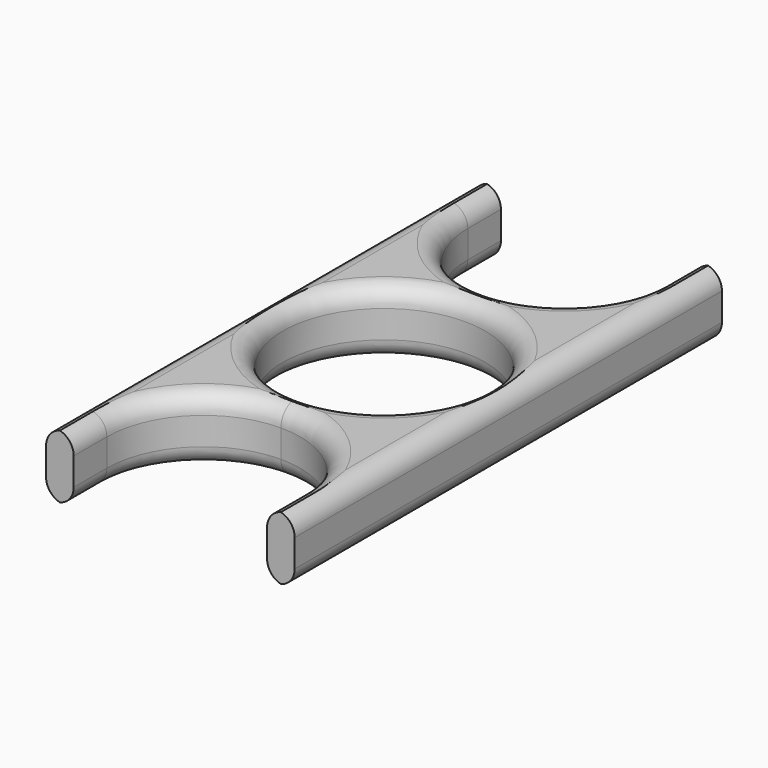
from build123d import *

# Parameters (mm, degrees)
F0_R          = 11
F1_DEPTH      = 7
F2_R          = 10.49999
F3_T1_DEPTH   = 9.50001
F3_T3_DEPTH   = 2e-05
F3_T5_DEPTH   = 68
F3_T7_DEPTH   = 9.50001
F3_T10_ANGLE  = 90
F3_T14_DEPTH  = 13
F3_S15_R      = 2
F3_T16_DEPTH  = 8
F3_T20_DEPTH  = 13
F3_S21_R      = 2
F3_T22_DEPTH  = 8
F3_T24_ANGLE  = 90
F3_T28_DEPTH  = 13
F3_S29_R      = 2
F3_T30_DEPTH  = 8
F3_T34_DEPTH  = 13
F3_S35_R      = 2
F3_T36_DEPTH  = 8
F3_T40_DEPTH  = 13
F3_S41_R      = 2
F3_T42_DEPTH  = 8
F3_T46_DEPTH  = 13
F3_S47_R      = 2
F3_T48_DEPTH  = 8
F3_T50_ANGLE  = 90
F3_T54_DEPTH  = 13
F3_S55_R      = 2
F3_T56_DEPTH  = 8
F3_T60_DEPTH  = 13
F3_S61_R      = 2
F3_T62_DEPTH  = 8
F3_T64_ANGLE  = 90
F3_T68_ANGLE  = 90
F3_T72_DEPTH  = 13
F3_S73_R      = 2
F3_T74_DEPTH  = 8
F3_T78_DEPTH  = 13
F3_S79_R      = 2
F3_T80_DEPTH  = 8
F3_T82_ANGLE  = 90
F3_T86_DEPTH  = 13
F3_S87_R      = 2
F3_T88_DEPTH  = 8
F3_T92_DEPTH  = 13
F3_S93_R      = 2
F3_T94_DEPTH  = 8
F3_T98_DEPTH  = 13
F3_S99_R      = 2
F3_T100_DEPTH = 8
F3_T104_DEPTH = 13
F3_S105_R     = 2
F3_T106_DEPTH = 8
F3_T108_ANGLE = 90
F3_T112_DEPTH = 13
F3_S113_R     = 2
F3_T114_DEPTH = 8
F3_T118_DEPTH = 13
F3_S119_R     = 2
F3_T120_DEPTH = 8
F3_T122_ANGLE = 90


# Not quite as in the source:
# - a fillet or chamfer that OpenCascade refuses, or shapes differently, is made with other operations: its cross-section is extruded or revolved along the edge and cut away or added
# - a fillet or chamfer is up to 0.001 mm smaller than in the source, because OpenCascade refuses the exact size


with BuildPart() as f1:
    # F0 (on Top) → F1 (new body)
    with BuildSketch(Plane.XY):
        Polygon((13.5, -29), (13.5, 29), (10.5, 29), (10.5, 14), (-10.5, 14), (-10.5, 29), (-13.5, 29), (-13.5, -29), (-10.5, -29), (-10.5, -14), (10.5, -14), (10.5, -29), align=None)
        Circle(F0_R, mode=Mode.SUBTRACT)
    extrude(amount=F1_DEPTH)

    # F2 (radius 10.5 in the source; OpenCascade refuses exactly that, so slightly less here)
    f2_edges = [f1.edges().sort_by_distance(p)[0] for p in [
        (-10.5, -14, 3.5),
        (10.5, -14, 3.5),
        (-10.5, 14, 3.5),
        (10.5, 14, 3.5),
    ]]
    fillet(f2_edges, radius=F2_R)

    # F3: fillet of radius 2 on 34 edges, made by hand

    # F3_s2 → F3_t1 (cut)
    with BuildSketch(Plane.XZ.offset(-34)):
        with BuildLine():
            ThreePointArc((10.5, 5), (11.0857864376, 6.4142135624), (12.5, 7))
            Line((12.5, 7), (10.5, 7))
            Line((10.5, 7), (10.5, 5))
        make_face()
        with BuildLine():
            ThreePointArc((-12.5, 7), (-11.0857864376, 6.4142135624), (-10.5, 5))
            Line((-10.5, 5), (-10.5, 7))
            Line((-10.5, 7), (-12.5, 7))
        make_face()
        with BuildLine():
            ThreePointArc((10.5, 2), (11.0857864376, 0.5857864376), (12.5, 0))
            Line((12.5, 0), (10.5, 0))
            Line((10.5, 0), (10.5, 2))
        make_face()
        with BuildLine():
            ThreePointArc((-12.5, 0), (-11.0857864376, 0.5857864376), (-10.5, 2))
            Line((-10.5, 2), (-10.5, 0))
            Line((-10.5, 0), (-12.5, 0))
        make_face()
    extrude(amount=F3_T1_DEPTH, mode=Mode.SUBTRACT)

    # F3_s4 → F3_t3 (cut)
    with BuildSketch(Plane.YZ.offset(-1e-05)):
        with BuildLine():
            ThreePointArc((12, 7), (13.4142135624, 6.4142135624), (14, 5))
            Line((14, 5), (14, 7))
            Line((14, 7), (12, 7))
        make_face()
        with BuildLine():
            ThreePointArc((-12, 7), (-13.4142135624, 6.4142135624), (-14, 5))
            Line((-14, 5), (-14, 7))
            Line((-14, 7), (-12, 7))
        make_face()
        with BuildLine():
            ThreePointArc((12, 0), (13.4142135624, 0.5857864376), (14, 2))
            Line((14, 2), (14, 0))
            Line((14, 0), (12, 0))
        make_face()
        with BuildLine():
            ThreePointArc((-12, 0), (-13.4142135624, 0.5857864376), (-14, 2))
            Line((-14, 2), (-14, 0))
            Line((-14, 0), (-12, 0))
        make_face()
    extrude(amount=F3_T3_DEPTH, mode=Mode.SUBTRACT)

    # F3_s6 → F3_t5 (cut)
    with BuildSketch(Plane.XZ.offset(-34)):
        with BuildLine():
            ThreePointArc((11.5, 7), (12.9142135624, 6.4142135624), (13.5, 5))
            Line((13.5, 5), (13.5, 7))
            Line((13.5, 7), (11.5, 7))
        make_face()
        with BuildLine():
            ThreePointArc((-11.5, 7), (-12.9142135624, 6.4142135624), (-13.5, 5))
            Line((-13.5, 5), (-13.5, 7))
            Line((-13.5, 7), (-11.5, 7))
        make_face()
        with BuildLine():
            ThreePointArc((11.5, 0), (12.9142135624, 0.5857864376), (13.5, 2))
            Line((13.5, 2), (13.5, 0))
            Line((13.5, 0), (11.5, 0))
        make_face()
        with BuildLine():
            ThreePointArc((-11.5, 0), (-12.9142135624, 0.5857864376), (-13.5, 2))
            Line((-13.5, 2), (-13.5, 0))
            Line((-13.5, 0), (-11.5, 0))
        make_face()
    extrude(amount=F3_T5_DEPTH, mode=Mode.SUBTRACT)

    # F3_s8 → F3_t7 (cut)
    with BuildSketch(Plane.XZ.offset(24.49999)):
        with BuildLine():
            ThreePointArc((12.5, 7), (11.0857864376, 6.4142135624), (10.5, 5))
            Line((10.5, 5), (10.5, 7))
            Line((10.5, 7), (12.5, 7))
        make_face()
        with BuildLine():
            ThreePointArc((-12.5, 7), (-11.0857864376, 6.4142135624), (-10.5, 5))
            Line((-10.5, 5), (-10.5, 7))
            Line((-10.5, 7), (-12.5, 7))
        make_face()
        with BuildLine():
            ThreePointArc((12.5, 0), (11.0857864376, 0.5857864376), (10.5, 2))
            Line((10.5, 2), (10.5, 0))
            Line((10.5, 0), (12.5, 0))
        make_face()
        with BuildLine():
            ThreePointArc((-12.5, 0), (-11.0857864376, 0.5857864376), (-10.5, 2))
            Line((-10.5, 2), (-10.5, 0))
            Line((-10.5, 0), (-12.5, 0))
        make_face()
    extrude(amount=F3_T7_DEPTH, mode=Mode.SUBTRACT)

    # F3_s9 → F3_t10 (revolve, cut)
    with BuildSketch(Plane.XZ.offset(-24.49999)):
        with BuildLine():
            ThreePointArc((10.5, 5), (11.0857864376, 6.4142135624), (12.5, 7))
            Line((12.5, 7), (10.5, 7))
            Line((10.5, 7), (10.5, 5))
        make_face()
    revolve(axis=Axis((1e-05, 24.49999, 7), (0, 0, -1)), revolution_arc=F3_T10_ANGLE, mode=Mode.SUBTRACT)


with BuildPart() as f3_tool12:
    # F3_s13 → F3_t14 (new body)
    with BuildSketch(Plane.YZ.offset(18.5)):
        with BuildLine():
            ThreePointArc((29, 5), (28.4142135624, 6.4142135624), (27, 7))
            Line((27, 7), (29, 7))
            Line((29, 7), (29, 5))
        make_face()
    extrude(amount=-F3_T14_DEPTH)

    # F3_s15 → F3_t16 (cut, symmetric)
    with BuildSketch(Plane.XZ.offset(-28)):
        with Locations((12.5, 5)):
            Circle(F3_S15_R)
    extrude(amount=F3_T16_DEPTH, both=True, mode=Mode.SUBTRACT)


with BuildPart() as f1_1:
    add(f1.part)

    # F3_t11: cut F3_tool12
    add(f3_tool12.part, mode=Mode.SUBTRACT)


with BuildPart() as f3_tool18:
    # F3_s19 → F3_t20 (new body)
    with BuildSketch(Plane.YZ.offset(18.5)):
        with BuildLine():
            ThreePointArc((29, 5), (28.4142135624, 6.4142135624), (27, 7))
            Line((27, 7), (29, 7))
            Line((29, 7), (29, 5))
        make_face()
    extrude(amount=-F3_T20_DEPTH)

    # F3_s21 → F3_t22 (cut, symmetric)
    with BuildSketch(Plane.XZ.offset(-28)):
        with Locations((11.5, 5)):
            Circle(F3_S21_R)
    extrude(amount=F3_T22_DEPTH, both=True, mode=Mode.SUBTRACT)


with BuildPart() as f1_2:
    add(f1_1.part)

    # F3_t17: cut F3_tool18
    add(f3_tool18.part, mode=Mode.SUBTRACT)

    # F3_s23 → F3_t24 (revolve, cut)
    with BuildSketch(Plane.YZ.offset(-1e-05)):
        with BuildLine():
            ThreePointArc((12, 7), (13.4142135624, 6.4142135624), (14, 5))
            Line((14, 5), (14, 7))
            Line((14, 7), (12, 7))
        make_face()
    revolve(axis=Axis((-1e-05, 24.49999, 7), (0, 0, -1)), revolution_arc=F3_T24_ANGLE, mode=Mode.SUBTRACT)


with BuildPart() as f3_tool26:
    # F3_s27 → F3_t28 (new body)
    with BuildSketch(Plane.YZ.offset(5.5)):
        with BuildLine():
            ThreePointArc((-27, 7), (-28.4142135624, 6.4142135624), (-29, 5))
            Line((-29, 5), (-29, 7))
            Line((-29, 7), (-27, 7))
        make_face()
    extrude(amount=F3_T28_DEPTH)

    # F3_s29 → F3_t30 (cut, symmetric)
    with BuildSketch(Plane.XZ.offset(28)):
        with Locations((12.5, 5)):
            Circle(F3_S29_R)
    extrude(amount=F3_T30_DEPTH, both=True, mode=Mode.SUBTRACT)


with BuildPart() as f1_3:
    add(f1_2.part)

    # F3_t25: cut F3_tool26
    add(f3_tool26.part, mode=Mode.SUBTRACT)


with BuildPart() as f3_tool32:
    # F3_s33 → F3_t34 (new body)
    with BuildSketch(Plane.YZ.offset(5.5)):
        with BuildLine():
            ThreePointArc((-27, 7), (-28.4142135624, 6.4142135624), (-29, 5))
            Line((-29, 5), (-29, 7))
            Line((-29, 7), (-27, 7))
        make_face()
    extrude(amount=F3_T34_DEPTH)

    # F3_s35 → F3_t36 (cut, symmetric)
    with BuildSketch(Plane.XZ.offset(28)):
        with Locations((11.5, 5)):
            Circle(F3_S35_R)
    extrude(amount=F3_T36_DEPTH, both=True, mode=Mode.SUBTRACT)


with BuildPart() as f1_4:
    add(f1_3.part)

    # F3_t31: cut F3_tool32
    add(f3_tool32.part, mode=Mode.SUBTRACT)


with BuildPart() as f3_tool38:
    # F3_s39 → F3_t40 (new body)
    with BuildSketch(Plane.YZ.offset(-5.5)):
        with BuildLine():
            ThreePointArc((27, 7), (28.4142135624, 6.4142135624), (29, 5))
            Line((29, 5), (29, 7))
            Line((29, 7), (27, 7))
        make_face()
    extrude(amount=-F3_T40_DEPTH)

    # F3_s41 → F3_t42 (cut, symmetric)
    with BuildSketch(Plane.XZ.offset(-28)):
        with Locations((-12.5, 5)):
            Circle(F3_S41_R)
    extrude(amount=F3_T42_DEPTH, both=True, mode=Mode.SUBTRACT)


with BuildPart() as f1_5:
    add(f1_4.part)

    # F3_t37: cut F3_tool38
    add(f3_tool38.part, mode=Mode.SUBTRACT)


with BuildPart() as f3_tool44:
    # F3_s45 → F3_t46 (new body)
    with BuildSketch(Plane.YZ.offset(-5.5)):
        with BuildLine():
            ThreePointArc((27, 7), (28.4142135624, 6.4142135624), (29, 5))
            Line((29, 5), (29, 7))
            Line((29, 7), (27, 7))
        make_face()
    extrude(amount=-F3_T46_DEPTH)

    # F3_s47 → F3_t48 (cut, symmetric)
    with BuildSketch(Plane.XZ.offset(-28)):
        with Locations((-11.5, 5)):
            Circle(F3_S47_R)
    extrude(amount=F3_T48_DEPTH, both=True, mode=Mode.SUBTRACT)


with BuildPart() as f1_6:
    add(f1_5.part)

    # F3_t43: cut F3_tool44
    add(f3_tool44.part, mode=Mode.SUBTRACT)

    # F3_s49 → F3_t50 (revolve, cut)
    with BuildSketch(Plane.YZ.offset(1e-05)):
        with BuildLine():
            ThreePointArc((-12, 7), (-13.4142135624, 6.4142135624), (-14, 5))
            Line((-14, 5), (-14, 7))
            Line((-14, 7), (-12, 7))
        make_face()
    revolve(axis=Axis((1e-05, -24.49999, 7), (0, 0, -1)), revolution_arc=F3_T50_ANGLE, mode=Mode.SUBTRACT)


with BuildPart() as f3_tool52:
    # F3_s53 → F3_t54 (new body)
    with BuildSketch(Plane.YZ.offset(-18.5)):
        with BuildLine():
            ThreePointArc((-27, 7), (-28.4142135624, 6.4142135624), (-29, 5))
            Line((-29, 5), (-29, 7))
            Line((-29, 7), (-27, 7))
        make_face()
    extrude(amount=F3_T54_DEPTH)

    # F3_s55 → F3_t56 (cut, symmetric)
    with BuildSketch(Plane.XZ.offset(28)):
        with Locations((-12.5, 5)):
            Circle(F3_S55_R)
    extrude(amount=F3_T56_DEPTH, both=True, mode=Mode.SUBTRACT)


with BuildPart() as f1_7:
    add(f1_6.part)

    # F3_t51: cut F3_tool52
    add(f3_tool52.part, mode=Mode.SUBTRACT)


with BuildPart() as f3_tool58:
    # F3_s59 → F3_t60 (new body)
    with BuildSketch(Plane.YZ.offset(-18.5)):
        with BuildLine():
            ThreePointArc((-27, 7), (-28.4142135624, 6.4142135624), (-29, 5))
            Line((-29, 5), (-29, 7))
            Line((-29, 7), (-27, 7))
        make_face()
    extrude(amount=F3_T60_DEPTH)

    # F3_s61 → F3_t62 (cut, symmetric)
    with BuildSketch(Plane.XZ.offset(28)):
        with Locations((-11.5, 5)):
            Circle(F3_S61_R)
    extrude(amount=F3_T62_DEPTH, both=True, mode=Mode.SUBTRACT)


with BuildPart() as f1_8:
    add(f1_7.part)

    # F3_t57: cut F3_tool58
    add(f3_tool58.part, mode=Mode.SUBTRACT)

    # F3_s63 → F3_t64 (revolve, cut)
    with BuildSketch(Plane.XZ.offset(24.49999)):
        with BuildLine():
            ThreePointArc((-12.5, 7), (-11.0857864376, 6.4142135624), (-10.5, 5))
            Line((-10.5, 5), (-10.5, 7))
            Line((-10.5, 7), (-12.5, 7))
        make_face()
    revolve(axis=Axis((-1e-05, -24.49999, 7), (0, 0, -1)), revolution_arc=F3_T64_ANGLE, mode=Mode.SUBTRACT)

    # F3_s65 → F3_t66 (revolve, cut)
    with BuildSketch(Plane.XZ):
        with BuildLine():
            ThreePointArc((13, 7), (11.5857864376, 6.4142135624), (11, 5))
            Line((11, 5), (11, 7))
            Line((11, 7), (13, 7))
        make_face()
    revolve(axis=Axis((0, 0, 7), (0, 0, 1)), mode=Mode.SUBTRACT)

    # F3_s67 → F3_t68 (revolve, cut)
    with BuildSketch(Plane.XZ.offset(-24.49999)):
        with BuildLine():
            ThreePointArc((12.5, 0), (11.0857864376, 0.5857864376), (10.5, 2))
            Line((10.5, 2), (10.5, 0))
            Line((10.5, 0), (12.5, 0))
        make_face()
    revolve(axis=Axis((1e-05, 24.49999, 0), (0, 0, -1)), revolution_arc=F3_T68_ANGLE, mode=Mode.SUBTRACT)


with BuildPart() as f3_tool70:
    # F3_s71 → F3_t72 (new body)
    with BuildSketch(Plane.YZ.offset(18.5)):
        with BuildLine():
            ThreePointArc((27, 0), (28.4142135624, 0.5857864376), (29, 2))
            Line((29, 2), (29, 0))
            Line((29, 0), (27, 0))
        make_face()
    extrude(amount=-F3_T72_DEPTH)

    # F3_s73 → F3_t74 (cut, symmetric)
    with BuildSketch(Plane.XZ.offset(-28)):
        with Locations((11.5, 2)):
            Circle(F3_S73_R)
    extrude(amount=F3_T74_DEPTH, both=True, mode=Mode.SUBTRACT)


with BuildPart() as f1_9:
    add(f1_8.part)

    # F3_t69: cut F3_tool70
    add(f3_tool70.part, mode=Mode.SUBTRACT)


with BuildPart() as f3_tool76:
    # F3_s77 → F3_t78 (new body)
    with BuildSketch(Plane.YZ.offset(18.5)):
        with BuildLine():
            ThreePointArc((27, 0), (28.4142135624, 0.5857864376), (29, 2))
            Line((29, 2), (29, 0))
            Line((29, 0), (27, 0))
        make_face()
    extrude(amount=-F3_T78_DEPTH)

    # F3_s79 → F3_t80 (cut, symmetric)
    with BuildSketch(Plane.XZ.offset(-28)):
        with Locations((12.5, 2)):
            Circle(F3_S79_R)
    extrude(amount=F3_T80_DEPTH, both=True, mode=Mode.SUBTRACT)


with BuildPart() as f1_10:
    add(f1_9.part)

    # F3_t75: cut F3_tool76
    add(f3_tool76.part, mode=Mode.SUBTRACT)

    # F3_s81 → F3_t82 (revolve, cut)
    with BuildSketch(Plane.YZ.offset(-1e-05)):
        with BuildLine():
            ThreePointArc((12, 0), (13.4142135624, 0.5857864376), (14, 2))
            Line((14, 2), (14, 0))
            Line((14, 0), (12, 0))
        make_face()
    revolve(axis=Axis((-1e-05, 24.49999, 0), (0, 0, -1)), revolution_arc=F3_T82_ANGLE, mode=Mode.SUBTRACT)


with BuildPart() as f3_tool84:
    # F3_s85 → F3_t86 (new body)
    with BuildSketch(Plane.YZ.offset(5.5)):
        with BuildLine():
            ThreePointArc((-27, 0), (-28.4142135624, 0.5857864376), (-29, 2))
            Line((-29, 2), (-29, 0))
            Line((-29, 0), (-27, 0))
        make_face()
    extrude(amount=F3_T86_DEPTH)

    # F3_s87 → F3_t88 (cut, symmetric)
    with BuildSketch(Plane.XZ.offset(28)):
        with Locations((11.5, 2)):
            Circle(F3_S87_R)
    extrude(amount=F3_T88_DEPTH, both=True, mode=Mode.SUBTRACT)


with BuildPart() as f1_11:
    add(f1_10.part)

    # F3_t83: cut F3_tool84
    add(f3_tool84.part, mode=Mode.SUBTRACT)


with BuildPart() as f3_tool90:
    # F3_s91 → F3_t92 (new body)
    with BuildSketch(Plane.YZ.offset(5.5)):
        with BuildLine():
            ThreePointArc((-27, 0), (-28.4142135624, 0.5857864376), (-29, 2))
            Line((-29, 2), (-29, 0))
            Line((-29, 0), (-27, 0))
        make_face()
    extrude(amount=F3_T92_DEPTH)

    # F3_s93 → F3_t94 (cut, symmetric)
    with BuildSketch(Plane.XZ.offset(28)):
        with Locations((12.5, 2)):
            Circle(F3_S93_R)
    extrude(amount=F3_T94_DEPTH, both=True, mode=Mode.SUBTRACT)


with BuildPart() as f1_12:
    add(f1_11.part)

    # F3_t89: cut F3_tool90
    add(f3_tool90.part, mode=Mode.SUBTRACT)


with BuildPart() as f3_tool96:
    # F3_s97 → F3_t98 (new body)
    with BuildSketch(Plane.YZ.offset(-5.5)):
        with BuildLine():
            ThreePointArc((27, 0), (28.4142135624, 0.5857864376), (29, 2))
            Line((29, 2), (29, 0))
            Line((29, 0), (27, 0))
        make_face()
    extrude(amount=-F3_T98_DEPTH)

    # F3_s99 → F3_t100 (cut, symmetric)
    with BuildSketch(Plane.XZ.offset(-28)):
        with Locations((-11.5, 2)):
            Circle(F3_S99_R)
    extrude(amount=F3_T100_DEPTH, both=True, mode=Mode.SUBTRACT)


with BuildPart() as f1_13:
    add(f1_12.part)

    # F3_t95: cut F3_tool96
    add(f3_tool96.part, mode=Mode.SUBTRACT)


with BuildPart() as f3_tool102:
    # F3_s103 → F3_t104 (new body)
    with BuildSketch(Plane.YZ.offset(-5.5)):
        with BuildLine():
            ThreePointArc((27, 0), (28.4142135624, 0.5857864376), (29, 2))
            Line((29, 2), (29, 0))
            Line((29, 0), (27, 0))
        make_face()
    extrude(amount=-F3_T104_DEPTH)

    # F3_s105 → F3_t106 (cut, symmetric)
    with BuildSketch(Plane.XZ.offset(-28)):
        with Locations((-12.5, 2)):
            Circle(F3_S105_R)
    extrude(amount=F3_T106_DEPTH, both=True, mode=Mode.SUBTRACT)


with BuildPart() as f1_14:
    add(f1_13.part)

    # F3_t101: cut F3_tool102
    add(f3_tool102.part, mode=Mode.SUBTRACT)

    # F3_s107 → F3_t108 (revolve, cut)
    with BuildSketch(Plane.YZ.offset(1e-05)):
        with BuildLine():
            ThreePointArc((-12, 0), (-13.4142135624, 0.5857864376), (-14, 2))
            Line((-14, 2), (-14, 0))
            Line((-14, 0), (-12, 0))
        make_face()
    revolve(axis=Axis((1e-05, -24.49999, 0), (0, 0, -1)), revolution_arc=F3_T108_ANGLE, mode=Mode.SUBTRACT)


with BuildPart() as f3_tool110:
    # F3_s111 → F3_t112 (new body)
    with BuildSketch(Plane.YZ.offset(-18.5)):
        with BuildLine():
            ThreePointArc((-27, 0), (-28.4142135624, 0.5857864376), (-29, 2))
            Line((-29, 2), (-29, 0))
            Line((-29, 0), (-27, 0))
        make_face()
    extrude(amount=F3_T112_DEPTH)

    # F3_s113 → F3_t114 (cut, symmetric)
    with BuildSketch(Plane.XZ.offset(28)):
        with Locations((-11.5, 2)):
            Circle(F3_S113_R)
    extrude(amount=F3_T114_DEPTH, both=True, mode=Mode.SUBTRACT)


with BuildPart() as f1_15:
    add(f1_14.part)

    # F3_t109: cut F3_tool110
    add(f3_tool110.part, mode=Mode.SUBTRACT)


with BuildPart() as f3_tool116:
    # F3_s117 → F3_t118 (new body)
    with BuildSketch(Plane.YZ.offset(-18.5)):
        with BuildLine():
            ThreePointArc((-27, 0), (-28.4142135624, 0.5857864376), (-29, 2))
            Line((-29, 2), (-29, 0))
            Line((-29, 0), (-27, 0))
        make_face()
    extrude(amount=F3_T118_DEPTH)

    # F3_s119 → F3_t120 (cut, symmetric)
    with BuildSketch(Plane.XZ.offset(28)):
        with Locations((-12.5, 2)):
            Circle(F3_S119_R)
    extrude(amount=F3_T120_DEPTH, both=True, mode=Mode.SUBTRACT)


with BuildPart() as f1_16:
    add(f1_15.part)

    # F3_t115: cut F3_tool116
    add(f3_tool116.part, mode=Mode.SUBTRACT)

    # F3_s121 → F3_t122 (revolve, cut)
    with BuildSketch(Plane.XZ.offset(24.49999)):
        with BuildLine():
            ThreePointArc((-12.5, 0), (-11.0857864376, 0.5857864376), (-10.5, 2))
            Line((-10.5, 2), (-10.5, 0))
            Line((-10.5, 0), (-12.5, 0))
        make_face()
    revolve(axis=Axis((-1e-05, -24.49999, 0), (0, 0, -1)), revolution_arc=F3_T122_ANGLE, mode=Mode.SUBTRACT)

    # F3_s123 → F3_t124 (revolve, cut)
    with BuildSketch(Plane.XZ):
        with BuildLine():
            ThreePointArc((13, 0), (11.5857864376, 0.5857864376), (11, 2))
            Line((11, 2), (11, 0))
            Line((11, 0), (13, 0))
        make_face()
    revolve(axis=Axis((0, 0, 0), (0, 0, 1)), mode=Mode.SUBTRACT)


solid = f1_16.part
